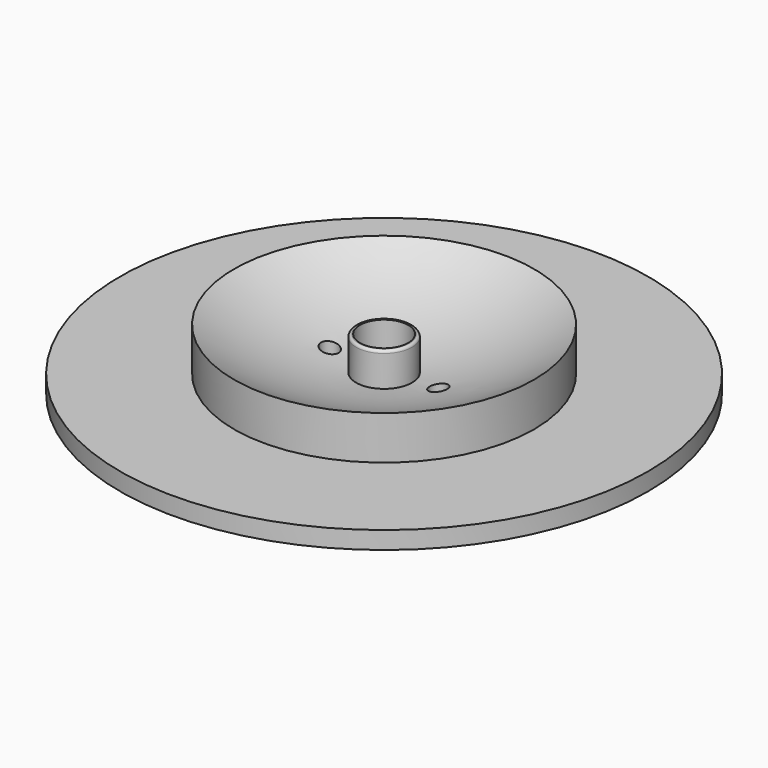
from build123d import *

# Parameters (mm, degrees)
F2_R          = 3.175
F2_R_2        = 2.75
F3_DEPTH      = 6
F3_DEPTH_BACK = 5
F4_R          = 0.3
F5_R          = 2.75
F6_DEPTH      = 6.966563666
F8_D          = 2


with BuildPart() as f1:
    # F0 (on Front) → F1 (revolve)
    with BuildSketch(Plane.XZ):
        Polygon((0, 2), (0, 0), (30, 0), (30, 2), (17.0486500744, 2), align=None)
        with BuildLine():
            ThreePointArc((17.0486500744, 6.965563649), (8.8785315808, 3.2666573852), (1.21e-08, 2))
            Line((1.21e-08, 2), (17.0486500744, 2))
            Line((17.0486500744, 2), (17.0486500744, 6.965563649))
        make_face()
    revolve(axis=Axis((0, 0, 32.75), (0, 0, -1)))

    # F2 (on Top) → F3 (join, two sides)
    with BuildSketch(Plane.XY) as f3_sk:
        Circle(F2_R)
        Circle(F2_R_2, mode=Mode.SUBTRACT)
    extrude(amount=F3_DEPTH)
    extrude(f3_sk.sketch, amount=-F3_DEPTH_BACK)

    # F4
    f4_edges = [f1.edges().sort_by_distance(p)[0] for p in [
        (-3.175, 0, 6),
    ]]
    fillet(f4_edges, radius=F4_R)

    # F5 (on face) → F6 (cut, through all)
    with BuildSketch(Plane(origin=(0, 0, 0), x_dir=(1, 0, 0), z_dir=(0, 0, -1))):
        Circle(F5_R)
    extrude(amount=-F6_DEPTH, mode=Mode.SUBTRACT)

    # F8 (through all)
    with Locations(Plane(origin=(0, 0, 0), x_dir=(1, 0, 0), z_dir=(0, 0, -1))):
        with Locations((-6.175, 0), (6.175, 0)):
            Hole(F8_D / 2)


solid = f1.part
